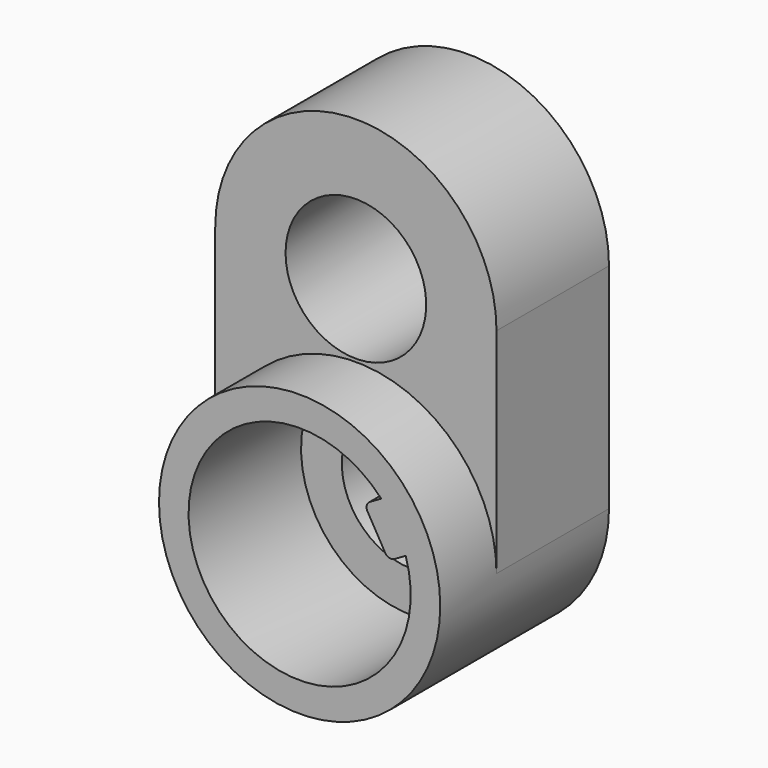
from build123d import *

# Parameters (mm, degrees)
F0_R     = 6.35
F0_R_2   = 3.175
F1_DEPTH = 3.175
F2_R     = 6.35
F2_R_2   = 5.0165
F3_DEPTH = 6.35
F4_R     = 3.175
F5_DEPTH = 6.35
F7_DEPTH = 6.35
F8_R     = 0.3048


# Not quite as in the source:
# - a feature names something its author has since deleted; it is built from what else it names


with BuildPart() as f1:
    # F0 (on Front) → F1 (new body)
    with BuildSketch(Plane.XZ):
        Circle(F0_R)
        Circle(F0_R_2, mode=Mode.SUBTRACT)
    extrude(amount=F1_DEPTH)

    # F2 (on face) → F3 (join)
    with BuildSketch(Plane.XZ.offset(3.175)):
        Circle(F2_R)
        Circle(F2_R_2, mode=Mode.SUBTRACT)
    extrude(amount=F3_DEPTH)

    # F4 (on face) → F5 (join)
    with BuildSketch(Plane(origin=(0, 0, 0), x_dir=(-1, 0, 0), z_dir=(0, 1, 0))):
        with BuildLine():
            ThreePointArc((-6.35, 9.652), (-5.7675394704, 6.9953125029), (-4.1270115096, 4.826))
            ThreePointArc((-4.1270115096, 4.826), (0, 6.35), (4.1270115096, 4.826))
            ThreePointArc((4.1270115096, 4.826), (5.7675394704, 6.9953125029), (6.35, 9.652))
            ThreePointArc((6.35, 9.652), (0, 16.002), (-6.35, 9.652))
        make_face()
        with Locations((0, 9.652)):
            Circle(F4_R, mode=Mode.SUBTRACT)
        with BuildLine():
            Line((-6.35, 9.652), (-6.35, 0))
            ThreePointArc((-6.35, 0), (-5.7675394704, 2.6566874971), (-4.1270115096, 4.826))
            ThreePointArc((-4.1270115096, 4.826), (-5.7675394704, 6.9953125029), (-6.35, 9.652))
        make_face()
        with BuildLine():
            ThreePointArc((4.1270115096, 4.826), (5.7675394704, 2.6566874971), (6.35, 0))
            Line((6.35, 0), (6.35, 9.652))
            ThreePointArc((6.35, 9.652), (5.7675394704, 6.9953125029), (4.1270115096, 4.826))
        make_face()
    extrude(amount=-F5_DEPTH)

    # F6 (on face) → F7 (join, through all)
    with BuildSketch(Plane.XZ.offset(9.525)):
        with BuildLine():
            Line((4.0169846278, 1.0433785314), (4.7901794841, 1.4897827897))
            ThreePointArc((4.7901794841, 1.4897827897), (4.3444164381, 2.50825), (3.6852794841, 3.403525727))
            Line((3.6852794841, 3.403525727), (2.9120846278, 2.9571214686))
            Line((2.9120846278, 2.9571214686), (4.0169846278, 1.0433785314))
        make_face()
    extrude(amount=-F7_DEPTH)

    # F8
    f8_edges = [f1.edges().sort_by_distance(p)[0] for p in [
        (2.912085, -6.35, 2.957121),
        (4.016985, -6.35, 1.043379),
    ]]
    fillet(f8_edges, radius=F8_R)


solid = f1.part
